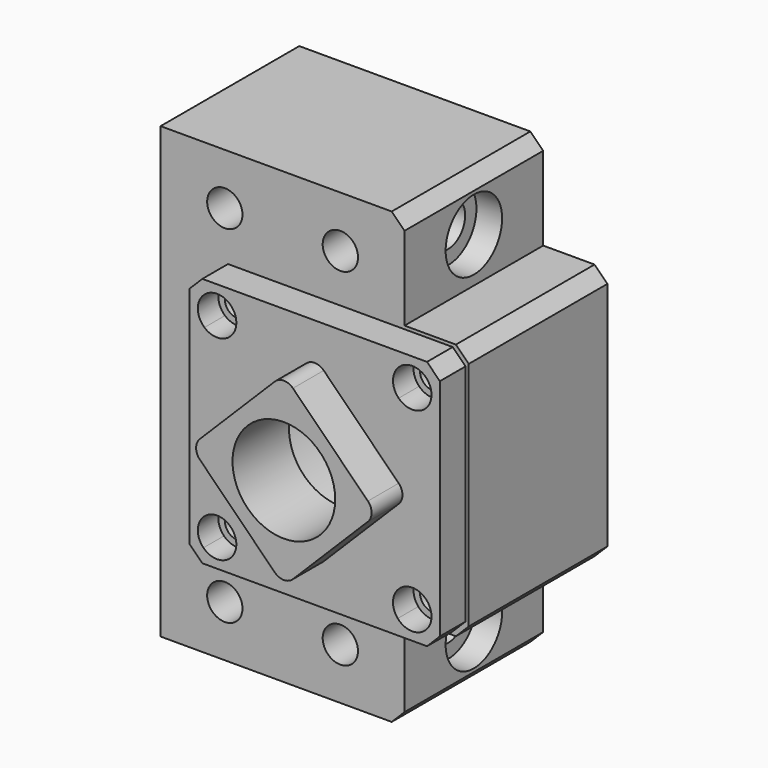
from build123d import *

# Parameters (mm, degrees)
F0_R        = 2.75
F0_R_2      = 16
F1_DEPTH    = 27
F2_R        = 3.3
F3_DEPTH    = 38
F4_R        = 5.5
F5_DEPTH    = 4
F6_SIZE     = 2
F7_R        = 16
F7_R_2      = 8
F8_DEPTH    = 5
F9_T1_DEPTH = 10.1433659759
F11_DEPTH   = 4
F12_R       = 2
F13_DEPTH   = 15
F14_R       = 8
F15_DEPTH   = 6


# Not quite as in the source:
# - a fillet or chamfer that OpenCascade refuses, or shapes differently, is made with other operations: its cross-section is extruded or revolved along the edge and cut away or added


with BuildPart() as f1:
    # F0 (on Front) → F1 (new body)
    with BuildSketch(Plane.XZ):
        Polygon((0, 70), (0, 0), (38, 0), (38, 15), (48, 15), (48, 55), (38, 55), (38, 70), align=None)
        with Locations((10, 8)):
            Circle(F0_R, mode=Mode.SUBTRACT)
        with Locations((28, 8)):
            Circle(F0_R, mode=Mode.SUBTRACT)
        with Locations((10, 62)):
            Circle(F0_R, mode=Mode.SUBTRACT)
        with Locations((28, 35)):
            Circle(F0_R_2, mode=Mode.SUBTRACT)
        with Locations((28, 62)):
            Circle(F0_R, mode=Mode.SUBTRACT)
    extrude(amount=F1_DEPTH)

    # F2 (on face) → F3 (cut)
    with BuildSketch(Plane.YZ.offset(38)):
        with Locations((-13.5, 62)):
            Circle(F2_R)
        with Locations((-13.5, 8)):
            Circle(F2_R)
    extrude(amount=-F3_DEPTH, mode=Mode.SUBTRACT)

    # F4 (on face) → F5 (cut)
    with BuildSketch(Plane.YZ.offset(38)):
        with Locations((-13.5, 62)):
            Circle(F4_R)
        with Locations((-13.5, 8)):
            Circle(F4_R)
    extrude(amount=-F5_DEPTH, mode=Mode.SUBTRACT)

    # F6
    f6_edges = [f1.edges().sort_by_distance(p)[0] for p in [
        (38, -13.5, 70),
        (48, -13.5, 55),
        (38, -13.5, 0),
        (48, -13.5, 15),
    ]]
    chamfer(f6_edges, length=F6_SIZE)

    # F7 (on face) → F8 (join)
    with BuildSketch(Plane.XZ.offset(27)):
        Polygon((8.5, 54.5), (8.5, 15.5), (46.5, 15.5), (47.5, 16.5), (47.5, 53.5), (46.5, 54.5), align=None)
        with Locations((28, 35)):
            Circle(F7_R, mode=Mode.SUBTRACT)
        Polygon((47.5, 54.5), (46.5, 54.5), (47.5, 53.5), align=None)
        Polygon((47.5, 16.5), (46.5, 15.5), (47.5, 15.5), align=None)
        with Locations((28, 35)):
            Circle(F7_R)
        with Locations((28, 35)):
            Circle(F7_R_2, mode=Mode.SUBTRACT)
    extrude(amount=F8_DEPTH)

    # F9: chamfer of 2 on 4 edges, made by hand

    # F9_s2 → F9_t1 (cut)
    with BuildSketch(Plane.XZ.offset(27)):
        Polygon((8.5, 17.5), (10.5, 15.5), (8.5, 15.5), align=None)
        Polygon((45.5, 15.5), (47.5, 17.5), (47.5, 15.5), align=None)
        Polygon((10.5, 54.5), (8.5, 52.5), (8.5, 54.5), align=None)
        Polygon((45.5, 54.5), (47.5, 52.5), (47.5, 54.5), align=None)
    extrude(amount=F9_T1_DEPTH, mode=Mode.SUBTRACT)

    # F10 (on face) → F11 (cut)
    with BuildSketch(Plane.XZ.offset(32)):
        with BuildLine():
            ThreePointArc((40.9386454151, 52.1709479885), (42.1050907163, 51.2264110599), (43.2027957955, 50.2027957955))
            Line((43.2027957955, 50.2027957955), (45.3241161391, 52.3241161391))
            ThreePointArc((45.3241161391, 52.3241161391), (43.0980808231, 53.2009677009), (40.9386454151, 52.1709479885))
        make_face()
        with BuildLine():
            ThreePointArc((41.081475452, 48.081475452), (43.0980808231, 47.2046238901), (45.1709479885, 47.9386454151))
            ThreePointArc((45.1709479885, 47.9386454151), (44.2264110599, 49.1050907163), (43.2027957955, 50.2027957955))
            Line((43.2027957955, 50.2027957955), (41.081475452, 48.081475452))
        make_face()
        with BuildLine():
            ThreePointArc((43.2027957955, 50.2027957955), (44.2264110599, 49.1050907163), (45.1709479885, 47.9386454151))
            ThreePointArc((45.1709479885, 47.9386454151), (45.9326727688, 48.9587010602), (46.2027957955, 50.2027957955))
            ThreePointArc((46.2027957955, 50.2027957955), (45.974434393, 51.3508460926), (45.3241161391, 52.3241161391))
            Line((45.3241161391, 52.3241161391), (43.2027957955, 50.2027957955))
        make_face()
        with BuildLine():
            Line((41.081475452, 48.081475452), (43.2027957955, 50.2027957955))
            ThreePointArc((43.2027957955, 50.2027957955), (42.1050907163, 51.2264110599), (40.9386454151, 52.1709479885))
            ThreePointArc((40.9386454151, 52.1709479885), (40.2046238901, 50.0980808231), (41.081475452, 48.081475452))
        make_face()
        with BuildLine():
            ThreePointArc((43.2027957955, 19.7972042045), (44.2264110599, 20.8949092837), (45.1709479885, 22.0613545849))
            ThreePointArc((45.1709479885, 22.0613545849), (43.0980808231, 22.7953761099), (41.081475452, 21.918524548))
            Line((41.081475452, 21.918524548), (43.2027957955, 19.7972042045))
        make_face()
        with BuildLine():
            ThreePointArc((46.2027957955, 19.7972042045), (45.9326727688, 21.0412989398), (45.1709479885, 22.0613545849))
            ThreePointArc((45.1709479885, 22.0613545849), (44.2264110599, 20.8949092837), (43.2027957955, 19.7972042045))
            Line((43.2027957955, 19.7972042045), (45.3241161391, 17.6758838609))
            ThreePointArc((45.3241161391, 17.6758838609), (45.974434393, 18.6491539074), (46.2027957955, 19.7972042045))
        make_face()
        with BuildLine():
            Line((45.3241161391, 17.6758838609), (43.2027957955, 19.7972042045))
            ThreePointArc((43.2027957955, 19.7972042045), (42.1050907163, 18.7735889401), (40.9386454151, 17.8290520115))
            ThreePointArc((40.9386454151, 17.8290520115), (43.0980808231, 16.7990322991), (45.3241161391, 17.6758838609))
        make_face()
        with BuildLine():
            ThreePointArc((40.9386454151, 17.8290520115), (42.1050907163, 18.7735889401), (43.2027957955, 19.7972042045))
            Line((43.2027957955, 19.7972042045), (41.081475452, 21.918524548))
            ThreePointArc((41.081475452, 21.918524548), (40.2046238901, 19.9019191769), (40.9386454151, 17.8290520115))
        make_face()
        with BuildLine():
            ThreePointArc((15.7972042045, 19.7972042045), (15.568842802, 20.9452545016), (14.918524548, 21.918524548))
            Line((14.918524548, 21.918524548), (12.7972042045, 19.7972042045))
            ThreePointArc((12.7972042045, 19.7972042045), (13.8949092837, 18.7735889401), (15.0613545849, 17.8290520115))
            ThreePointArc((15.0613545849, 17.8290520115), (15.6072265479, 18.7465975087), (15.7972042045, 19.7972042045))
        make_face()
        with BuildLine():
            Line((10.6758838609, 17.6758838609), (12.7972042045, 19.7972042045))
            ThreePointArc((12.7972042045, 19.7972042045), (11.7735889401, 20.8949092837), (10.8290520115, 22.0613545849))
            ThreePointArc((10.8290520115, 22.0613545849), (9.7990322991, 19.9019191769), (10.6758838609, 17.6758838609))
        make_face()
        with BuildLine():
            Line((12.7972042045, 19.7972042045), (14.918524548, 21.918524548))
            ThreePointArc((14.918524548, 21.918524548), (12.9019191769, 22.7953761099), (10.8290520115, 22.0613545849))
            ThreePointArc((10.8290520115, 22.0613545849), (11.7735889401, 20.8949092837), (12.7972042045, 19.7972042045))
        make_face()
        with BuildLine():
            ThreePointArc((10.6758838609, 17.6758838609), (12.9019191769, 16.7990322991), (15.0613545849, 17.8290520115))
            ThreePointArc((15.0613545849, 17.8290520115), (13.8949092837, 18.7735889401), (12.7972042045, 19.7972042045))
            Line((12.7972042045, 19.7972042045), (10.6758838609, 17.6758838609))
        make_face()
        with BuildLine():
            ThreePointArc((12.7972042045, 50.2027957955), (13.8949092837, 51.2264110599), (15.0613545849, 52.1709479885))
            ThreePointArc((15.0613545849, 52.1709479885), (12.9019191769, 53.2009677009), (10.6758838609, 52.3241161391))
            Line((10.6758838609, 52.3241161391), (12.7972042045, 50.2027957955))
        make_face()
        with BuildLine():
            ThreePointArc((10.8290520115, 47.9386454151), (12.9019191769, 47.2046238901), (14.918524548, 48.081475452))
            Line((14.918524548, 48.081475452), (12.7972042045, 50.2027957955))
            ThreePointArc((12.7972042045, 50.2027957955), (11.7735889401, 49.1050907163), (10.8290520115, 47.9386454151))
        make_face()
        with BuildLine():
            Line((12.7972042045, 50.2027957955), (14.918524548, 48.081475452))
            ThreePointArc((14.918524548, 48.081475452), (15.568842802, 49.0547454984), (15.7972042045, 50.2027957955))
            ThreePointArc((15.7972042045, 50.2027957955), (15.6072265479, 51.2534024913), (15.0613545849, 52.1709479885))
            ThreePointArc((15.0613545849, 52.1709479885), (13.8949092837, 51.2264110599), (12.7972042045, 50.2027957955))
        make_face()
        with BuildLine():
            ThreePointArc((10.8290520115, 47.9386454151), (11.7735889401, 49.1050907163), (12.7972042045, 50.2027957955))
            Line((12.7972042045, 50.2027957955), (10.6758838609, 52.3241161391))
            ThreePointArc((10.6758838609, 52.3241161391), (9.7990322991, 50.0980808231), (10.8290520115, 47.9386454151))
        make_face()
    extrude(amount=-F11_DEPTH, mode=Mode.SUBTRACT)

    # F12 (on face) → F13 (cut)
    with BuildSketch(Plane.XZ.offset(32)):
        with Locations((43.2027957955, 50.2027957955)):
            Circle(F12_R)
        with Locations((43.2027957955, 19.7972042045)):
            Circle(F12_R)
        with Locations((12.7972042045, 19.7972042045)):
            Circle(F12_R)
        with Locations((12.7972042045, 50.2027957955)):
            Circle(F12_R)
    extrude(amount=-F13_DEPTH, mode=Mode.SUBTRACT)

    # F14 (on face) → F15 (join)
    with BuildSketch(Plane.XZ.offset(32)):
        with BuildLine():
            Line((26.5857864376, 48.0857864376), (14.9142135624, 36.4142135624))
            ThreePointArc((14.9142135624, 36.4142135624), (14.3284271247, 35), (14.9142135624, 33.5857864376))
            Line((14.9142135624, 33.5857864376), (26.5857864376, 21.9142135624))
            ThreePointArc((26.5857864376, 21.9142135624), (28, 21.3284271247), (29.4142135624, 21.9142135624))
            Line((29.4142135624, 21.9142135624), (41.0857864376, 33.5857864376))
            ThreePointArc((41.0857864376, 33.5857864376), (41.6715728753, 35), (41.0857864376, 36.4142135624))
            Line((41.0857864376, 36.4142135624), (29.4142135624, 48.0857864376))
            ThreePointArc((29.4142135624, 48.0857864376), (28, 48.6715728753), (26.5857864376, 48.0857864376))
        make_face()
        with Locations((28, 35)):
            Circle(F14_R, mode=Mode.SUBTRACT)
    extrude(amount=F15_DEPTH)


solid = f1.part
